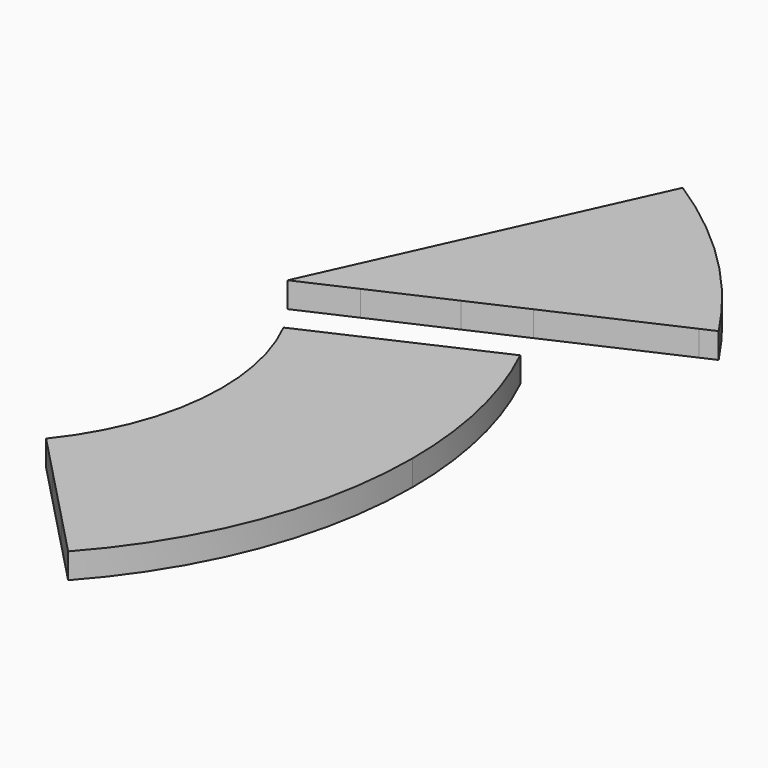
from build123d import *

# Parameters (mm, degrees)
F0_R        = 1.5044645314
F1_DEPTH    = 2.7
F2_DEPTH    = 0.9
F3_DEPTH    = 2.7
F4_DEPTH    = 0.9
F5_T1_DEPTH = 2.7
F6_DEPTH    = 0.9


# Not quite as in the source:
# - a fillet or chamfer that OpenCascade refuses, or shapes differently, is made with other operations: its cross-section is extruded or revolved along the edge and cut away or added


with BuildPart() as f1:
    # F0 (on Top) → F1 (new body)
    with BuildSketch(Plane.XY):
        with BuildLine():
            ThreePointArc((-2.9059050305, 19.7877668258), (-18.361479671, -7.928181651), (12.4102011034, -15.6839697964))
            Line((12.4102011034, -15.6839697964), (9.3065271924, -12.2254227754))
            ThreePointArc((9.3065271924, -12.2254227754), (-15.2699304913, -1.7034180964), (6.3836906961, 13.9757255095))
            Line((6.3836906961, 13.9757255095), (8.1864677167, 18.2477874364))
            ThreePointArc((8.1864677167, 18.2477874364), (5.5993809855, 19.2001805351), (2.9059050305, 19.7877668258))
            ThreePointArc((2.9059050305, 19.7877668258), (0, 18.1241204417), (-2.9059050305, 19.7877668258))
        make_face()
        with BuildLine():
            ThreePointArc((6.3836906961, 13.9757255095), (-15.2699304913, -1.7034180964), (9.3065271924, -12.2254227754))
            Line((9.3065271924, -12.2254227754), (7.9527661976, -10.7168731694))
            ThreePointArc((7.9527661976, -10.7168731694), (-13.2749249311, -1.3690247612), (5.5982117915, 12.114366903))
            Line((5.5982117915, 12.114366903), (6.3836906961, 13.9757255095))
        make_face()
        with BuildLine():
            ThreePointArc((5.5982117915, 12.114366903), (-13.2749249311, -1.3690247612), (7.9527661976, -10.7168731694))
            Line((7.9527661976, -10.7168731694), (6.0964799797, -8.6483397626))
            ThreePointArc((6.0964799797, -8.6483397626), (-10.5418803683, -0.9108276969), (4.5227579261, 9.5658512185))
            Line((4.5227579261, 9.5658512185), (5.5982117915, 12.114366903))
        make_face()
        with BuildLine():
            ThreePointArc((4.5227579261, 9.5658512185), (-10.5418803683, -0.9108276969), (6.0964799797, -8.6483397626))
            Line((6.0964799797, -8.6483397626), (4.7718042528, -7.1722010249))
            ThreePointArc((4.7718042528, -7.1722010249), (-8.5947223482, -0.5842355063), (3.7573171653, 7.7519772374))
            Line((3.7573171653, 7.7519772374), (4.5227579261, 9.5658512185))
        make_face()
        with BuildLine():
            ThreePointArc((3.7573171653, 7.7519772374), (-8.5947223482, -0.5842355063), (4.7718042528, -7.1722010249))
            Line((4.7718042528, -7.1722010249), (1.6593857385, -3.7039095455))
            ThreePointArc((1.6593857385, -3.7039095455), (-4.0546444127, 0.1799045205), (1.9809039535, 3.5423899386))
            Line((1.9809039535, 3.5423899386), (3.7573171653, 7.7519772374))
        make_face()
        with BuildLine():
            ThreePointArc((2.9059050305, 19.7877668258), (0, 20), (-2.9059050305, 19.7877668258))
            ThreePointArc((-2.9059050305, 19.7877668258), (0, 18.1241204417), (2.9059050305, 19.7877668258))
        make_face()
        with BuildLine():
            ThreePointArc((-3.157685128, 20.3174125427), (-3.043339046, 20.0471019762), (-2.9059050305, 19.7877668258))
            ThreePointArc((-2.9059050305, 19.7877668258), (0, 20), (2.9059050305, 19.7877668258))
            ThreePointArc((2.9059050305, 19.7877668258), (3.043339046, 20.0471019762), (3.157685128, 20.3174125427))
            ThreePointArc((3.157685128, 20.3174125427), (0, 20.5613284541), (-3.157685128, 20.3174125427))
        make_face()
        with BuildLine():
            ThreePointArc((3.3697074825, 21.4938279241), (-0.5976844127, 24.8101062388), (-3.157685128, 20.3174125427))
            ThreePointArc((-3.157685128, 20.3174125427), (0, 20.5613284541), (3.157685128, 20.3174125427))
            ThreePointArc((3.157685128, 20.3174125427), (3.3162783146, 20.8961435115), (3.3697074825, 21.4938279241))
        make_face()
        with Locations((0, 22.4330537021)):
            Circle(F0_R, mode=Mode.SUBTRACT)
        with BuildLine():
            ThreePointArc((13.8344540426, 6.6843318112), (13.1730545976, 7.9084159596), (12.4036340143, 9.0676498421))
            Line((12.4036340143, 9.0676498421), (10.5172175152, 8.21498609))
            ThreePointArc((10.5172175152, 8.21498609), (11.318131065, 7.0709101194), (11.995098321, 5.8493997121))
            Line((11.995098321, 5.8493997121), (13.8344540426, 6.6843318112))
        make_face()
        with BuildLine():
            ThreePointArc((11.995098321, 5.8493997121), (11.318131065, 7.0709101194), (10.5172175152, 8.21498609))
            Line((10.5172175152, 8.21498609), (7.9045951482, 7.0340759404))
            ThreePointArc((7.9045951482, 7.0340759404), (8.7683299388, 5.9226040621), (9.4768887451, 4.706317935))
            Line((9.4768887451, 4.706317935), (11.995098321, 5.8493997121))
        make_face()
        with BuildLine():
            ThreePointArc((9.4768887451, 4.706317935), (8.7683299388, 5.9226040621), (7.9045951482, 7.0340759404))
            Line((7.9045951482, 7.0340759404), (6.0058132946, 6.1758230253))
            ThreePointArc((6.0058132946, 6.1758230253), (6.9398340598, 5.1038501734), (7.6848114732, 3.8928467719))
            Line((7.6848114732, 3.8928467719), (9.4768887451, 4.706317935))
        make_face()
        with BuildLine():
            Line((6.0058132946, 6.1758230253), (7.9045951482, 7.0340759404))
            ThreePointArc((7.9045951482, 7.0340759404), (7.4001814409, 7.5629467428), (6.8604632985, 8.0557365971))
            Line((6.8604632985, 8.0557365971), (6.0058132946, 6.1758230253))
        make_face()
        with BuildLine():
            ThreePointArc((6.8604632985, 8.0557365971), (5.7414756731, 8.8879866049), (4.5227579261, 9.5658512185))
            Line((4.5227579261, 9.5658512185), (3.7573171653, 7.7519772374))
            ThreePointArc((3.7573171653, 7.7519772374), (4.9447694202, 7.0540654058), (6.0058132946, 6.1758230253))
            Line((6.0058132946, 6.1758230253), (6.8604632985, 8.0557365971))
        make_face()
        with BuildLine():
            ThreePointArc((8.0404414582, 10.6512516579), (6.8584540657, 11.4481207432), (5.5982117915, 12.114366903))
            Line((5.5982117915, 12.114366903), (4.5227579261, 9.5658512185))
            ThreePointArc((4.5227579261, 9.5658512185), (5.7414756731, 8.8879866049), (6.8604632985, 8.0557365971))
            Line((6.8604632985, 8.0557365971), (8.0404414582, 10.6512516579))
        make_face()
        with BuildLine():
            ThreePointArc((8.8939895289, 12.5287413845), (7.6730254156, 13.3115397829), (6.3836906961, 13.9757255095))
            Line((6.3836906961, 13.9757255095), (5.5982117915, 12.114366903))
            ThreePointArc((5.5982117915, 12.114366903), (6.8584540657, 11.4481207432), (8.0404414582, 10.6512516579))
            Line((8.0404414582, 10.6512516579), (8.8939895289, 12.5287413845))
        make_face()
        with BuildLine():
            Line((7.9045951482, 7.0340759404), (10.5172175152, 8.21498609))
            ThreePointArc((10.5172175152, 8.21498609), (9.3584466725, 9.514059943), (8.0404414582, 10.6512516579))
            Line((8.0404414582, 10.6512516579), (6.8604632985, 8.0557365971))
            ThreePointArc((6.8604632985, 8.0557365971), (7.4001814409, 7.5629467428), (7.9045951482, 7.0340759404))
        make_face()
        with BuildLine():
            Line((10.5172175152, 8.21498609), (12.4036340143, 9.0676498421))
            ThreePointArc((12.4036340143, 9.0676498421), (10.7885115198, 10.9398550999), (8.8939895289, 12.5287413845))
            Line((8.8939895289, 12.5287413845), (8.0404414582, 10.6512516579))
            ThreePointArc((8.0404414582, 10.6512516579), (9.3584466725, 9.514059943), (10.5172175152, 8.21498609))
        make_face()
        with BuildLine():
            Line((12.4036340143, 9.0676498421), (16.6976556484, 11.008555575))
            ThreePointArc((16.6976556484, 11.008555575), (14.070563524, 14.2133473227), (10.8394114429, 16.807949297))
            Line((10.8394114429, 16.807949297), (8.8939895289, 12.5287413845))
            ThreePointArc((8.8939895289, 12.5287413845), (10.7885115198, 10.9398550999), (12.4036340143, 9.0676498421))
        make_face()
        with BuildLine():
            ThreePointArc((10.8394114429, 16.807949297), (14.070563524, 14.2133473227), (16.6976556484, 11.008555575))
            Line((16.6976556484, 11.008555575), (17.2154603994, 11.2426042817))
            ThreePointArc((17.2154603994, 11.2426042817), (14.4679762691, 14.6097874889), (11.0741551061, 17.3242984413))
            Line((11.0741551061, 17.3242984413), (10.8394114429, 16.807949297))
        make_face()
    extrude(amount=-F1_DEPTH)

    # F0 (on Top) → F2 (join)
    with BuildSketch(Plane.XY):
        with BuildLine():
            ThreePointArc((-2.9059050305, 19.7877668258), (-18.361479671, -7.928181651), (12.4102011034, -15.6839697964))
            Line((12.4102011034, -15.6839697964), (9.3065271924, -12.2254227754))
            ThreePointArc((9.3065271924, -12.2254227754), (-15.2699304913, -1.7034180964), (6.3836906961, 13.9757255095))
            Line((6.3836906961, 13.9757255095), (8.1864677167, 18.2477874364))
            ThreePointArc((8.1864677167, 18.2477874364), (5.5993809855, 19.2001805351), (2.9059050305, 19.7877668258))
            ThreePointArc((2.9059050305, 19.7877668258), (0, 18.1241204417), (-2.9059050305, 19.7877668258))
        make_face()
        with BuildLine():
            ThreePointArc((6.3836906961, 13.9757255095), (-15.2699304913, -1.7034180964), (9.3065271924, -12.2254227754))
            Line((9.3065271924, -12.2254227754), (7.9527661976, -10.7168731694))
            ThreePointArc((7.9527661976, -10.7168731694), (-13.2749249311, -1.3690247612), (5.5982117915, 12.114366903))
            Line((5.5982117915, 12.114366903), (6.3836906961, 13.9757255095))
        make_face()
        with BuildLine():
            ThreePointArc((4.5227579261, 9.5658512185), (-10.5418803683, -0.9108276969), (6.0964799797, -8.6483397626))
            Line((6.0964799797, -8.6483397626), (4.7718042528, -7.1722010249))
            ThreePointArc((4.7718042528, -7.1722010249), (-8.5947223482, -0.5842355063), (3.7573171653, 7.7519772374))
            Line((3.7573171653, 7.7519772374), (4.5227579261, 9.5658512185))
        make_face()
        with BuildLine():
            ThreePointArc((3.7573171653, 7.7519772374), (-8.5947223482, -0.5842355063), (4.7718042528, -7.1722010249))
            Line((4.7718042528, -7.1722010249), (1.6593857385, -3.7039095455))
            ThreePointArc((1.6593857385, -3.7039095455), (-4.0546444127, 0.1799045205), (1.9809039535, 3.5423899386))
            Line((1.9809039535, 3.5423899386), (3.7573171653, 7.7519772374))
        make_face()
        with BuildLine():
            ThreePointArc((2.9059050305, 19.7877668258), (0, 20), (-2.9059050305, 19.7877668258))
            ThreePointArc((-2.9059050305, 19.7877668258), (0, 18.1241204417), (2.9059050305, 19.7877668258))
        make_face()
    extrude(amount=F2_DEPTH)

    # F0 (on Top) → F3 (join)
    with BuildSketch(Plane.XY):
        with BuildLine():
            Line((6.7113864418, -5.4007291543), (8.0821585416, -6.8293163715))
            ThreePointArc((8.0821585416, -6.8293163715), (9.9367857977, -3.6360881181), (10.5811553619, 0))
            ThreePointArc((10.5811553619, 0), (10.3013902205, 2.4170660555), (9.4768887451, 4.706317935))
            Line((9.4768887451, 4.706317935), (7.6848114732, 3.8928467719))
            ThreePointArc((7.6848114732, 3.8928467719), (8.3788968801, 2.00116727), (8.6145564813, 0))
            ThreePointArc((8.6145564813, 0), (8.1248446428, -2.8631246741), (6.7113864418, -5.4007291543))
        make_face()
        with BuildLine():
            Line((8.0821585416, -6.8293163715), (10.0042554899, -8.8324816906))
            ThreePointArc((10.0042554899, -8.8324816906), (12.4821464921, -4.721639511), (13.3453310458, 0))
            ThreePointArc((13.3453310458, 0), (13.0033922255, 3.0016081275), (11.995098321, 5.8493997121))
            Line((11.995098321, 5.8493997121), (9.4768887451, 4.706317935))
            ThreePointArc((9.4768887451, 4.706317935), (10.3013902205, 2.4170660555), (10.5811553619, 0))
            ThreePointArc((10.5811553619, 0), (9.9367857977, -3.6360881181), (8.0821585416, -6.8293163715))
        make_face()
        with BuildLine():
            Line((10.0042554899, -8.8324816906), (11.4065098197, -10.2938789654))
            ThreePointArc((11.4065098197, -10.2938789654), (14.3410149492, -5.5143177862), (15.3646480734, 0))
            ThreePointArc((15.3646480734, 0), (14.9772148291, 3.4286216448), (13.8344540426, 6.6843318112))
            Line((13.8344540426, 6.6843318112), (11.995098321, 5.8493997121))
            ThreePointArc((11.995098321, 5.8493997121), (13.0033922255, 3.0016081275), (13.3453310458, 0))
            ThreePointArc((13.3453310458, 0), (12.4821464921, -4.721639511), (10.0042554899, -8.8324816906))
        make_face()
        with BuildLine():
            Line((7.9527661976, -10.7168731694), (9.3065271924, -12.2254227754))
            ThreePointArc((9.3065271924, -12.2254227754), (10.4014513861, -11.3085020883), (11.4065098197, -10.2938789654))
            Line((11.4065098197, -10.2938789654), (10.0042554899, -8.8324816906))
            ThreePointArc((10.0042554899, -8.8324816906), (9.0278120152, -9.8283503672), (7.9527661976, -10.7168731694))
        make_face()
        with BuildLine():
            Line((6.0964799797, -8.6483397626), (7.9527661976, -10.7168731694))
            ThreePointArc((7.9527661976, -10.7168731694), (9.0278120152, -9.8283503672), (10.0042554899, -8.8324816906))
            Line((10.0042554899, -8.8324816906), (8.0821585416, -6.8293163715))
            ThreePointArc((8.0821585416, -6.8293163715), (7.1474232492, -7.8022554232), (6.0964799797, -8.6483397626))
        make_face()
        with BuildLine():
            Line((4.7718042528, -7.1722010249), (6.0964799797, -8.6483397626))
            ThreePointArc((6.0964799797, -8.6483397626), (7.1474232492, -7.8022554232), (8.0821585416, -6.8293163715))
            Line((8.0821585416, -6.8293163715), (6.7113864418, -5.4007291543))
            ThreePointArc((6.7113864418, -5.4007291543), (5.8095133427, -6.3608284122), (4.7718042528, -7.1722010249))
        make_face()
    extrude(amount=-F3_DEPTH)

    # F0 (on Top) → F4 (join)
    with BuildSketch(Plane.XY):
        with BuildLine():
            Line((10.0042554899, -8.8324816906), (11.4065098197, -10.2938789654))
            ThreePointArc((11.4065098197, -10.2938789654), (14.3410149492, -5.5143177862), (15.3646480734, 0))
            ThreePointArc((15.3646480734, 0), (14.9772148291, 3.4286216448), (13.8344540426, 6.6843318112))
            Line((13.8344540426, 6.6843318112), (11.995098321, 5.8493997121))
            ThreePointArc((11.995098321, 5.8493997121), (13.0033922255, 3.0016081275), (13.3453310458, 0))
            ThreePointArc((13.3453310458, 0), (12.4821464921, -4.721639511), (10.0042554899, -8.8324816906))
        make_face()
        with BuildLine():
            Line((8.0821585416, -6.8293163715), (10.0042554899, -8.8324816906))
            ThreePointArc((10.0042554899, -8.8324816906), (12.4821464921, -4.721639511), (13.3453310458, 0))
            ThreePointArc((13.3453310458, 0), (13.0033922255, 3.0016081275), (11.995098321, 5.8493997121))
            Line((11.995098321, 5.8493997121), (9.4768887451, 4.706317935))
            ThreePointArc((9.4768887451, 4.706317935), (10.3013902205, 2.4170660555), (10.5811553619, 0))
            ThreePointArc((10.5811553619, 0), (9.9367857977, -3.6360881181), (8.0821585416, -6.8293163715))
        make_face()
        with BuildLine():
            Line((6.7113864418, -5.4007291543), (8.0821585416, -6.8293163715))
            ThreePointArc((8.0821585416, -6.8293163715), (9.9367857977, -3.6360881181), (10.5811553619, 0))
            ThreePointArc((10.5811553619, 0), (10.3013902205, 2.4170660555), (9.4768887451, 4.706317935))
            Line((9.4768887451, 4.706317935), (7.6848114732, 3.8928467719))
            ThreePointArc((7.6848114732, 3.8928467719), (8.3788968801, 2.00116727), (8.6145564813, 0))
            ThreePointArc((8.6145564813, 0), (8.1248446428, -2.8631246741), (6.7113864418, -5.4007291543))
        make_face()
        with BuildLine():
            ThreePointArc((10.8394114429, 16.807949297), (14.070563524, 14.2133473227), (16.6976556484, 11.008555575))
            Line((16.6976556484, 11.008555575), (17.2154603994, 11.2426042817))
            ThreePointArc((17.2154603994, 11.2426042817), (14.4679762691, 14.6097874889), (11.0741551061, 17.3242984413))
            Line((11.0741551061, 17.3242984413), (10.8394114429, 16.807949297))
        make_face()
        with BuildLine():
            Line((6.0058132946, 6.1758230253), (7.9045951482, 7.0340759404))
            ThreePointArc((7.9045951482, 7.0340759404), (7.4001814409, 7.5629467428), (6.8604632985, 8.0557365971))
            Line((6.8604632985, 8.0557365971), (6.0058132946, 6.1758230253))
        make_face()
        with BuildLine():
            Line((7.9045951482, 7.0340759404), (10.5172175152, 8.21498609))
            ThreePointArc((10.5172175152, 8.21498609), (9.3584466725, 9.514059943), (8.0404414582, 10.6512516579))
            Line((8.0404414582, 10.6512516579), (6.8604632985, 8.0557365971))
            ThreePointArc((6.8604632985, 8.0557365971), (7.4001814409, 7.5629467428), (7.9045951482, 7.0340759404))
        make_face()
        with BuildLine():
            Line((10.5172175152, 8.21498609), (12.4036340143, 9.0676498421))
            ThreePointArc((12.4036340143, 9.0676498421), (10.7885115198, 10.9398550999), (8.8939895289, 12.5287413845))
            Line((8.8939895289, 12.5287413845), (8.0404414582, 10.6512516579))
            ThreePointArc((8.0404414582, 10.6512516579), (9.3584466725, 9.514059943), (10.5172175152, 8.21498609))
        make_face()
        with BuildLine():
            Line((12.4036340143, 9.0676498421), (16.6976556484, 11.008555575))
            ThreePointArc((16.6976556484, 11.008555575), (14.070563524, 14.2133473227), (10.8394114429, 16.807949297))
            Line((10.8394114429, 16.807949297), (8.8939895289, 12.5287413845))
            ThreePointArc((8.8939895289, 12.5287413845), (10.7885115198, 10.9398550999), (12.4036340143, 9.0676498421))
        make_face()
    extrude(amount=F4_DEPTH)

    # F5: fillet of radius 3 on 2 edges, made by hand

    # F5_s2 → F5_t1 (join)
    with BuildSketch(Plane.XY.offset(-2.7)):
        with BuildLine():
            ThreePointArc((3.3539587166, 21.8192345075), (4.0340965589, 20.1897997022), (5.5129894146, 19.2251644392))
            ThreePointArc((5.5129894146, 19.2251644392), (4.2188358916, 19.5499724736), (2.9059050305, 19.7877668258))
            ThreePointArc((2.9059050305, 19.7877668258), (3.2906213347, 20.768059539), (3.3539587166, 21.8192345075))
        make_face()
        with BuildLine():
            ThreePointArc((-3.3539587166, 21.8192345075), (-4.0340965589, 20.1897997022), (-5.5129894146, 19.2251644392))
            ThreePointArc((-5.5129894146, 19.2251644392), (-4.2188358916, 19.5499724736), (-2.9059050305, 19.7877668258))
            ThreePointArc((-2.9059050305, 19.7877668258), (-3.2906213347, 20.768059539), (-3.3539587166, 21.8192345075))
        make_face()
    extrude(amount=F5_T1_DEPTH)


with BuildPart() as f6:
    # F6 (new): a face of the model
    f6_faces = [f1.part.faces().sort_by_distance(p)[0] for p in [
        (11.5302934708, -1.5094822973, 0.9),
    ]]
    extrude(f6_faces, amount=F6_DEPTH)


with BuildPart() as f6b:
    # F6#2 (new): a face of the model
    f6_2_faces = [f1.part.faces().sort_by_distance(p)[0] for p in [
        (11.5759648362, 11.7245978836, 0.9),
    ]]
    extrude(f6_2_faces, amount=F6_DEPTH)


solid = Compound([f6.part, f6b.part])
